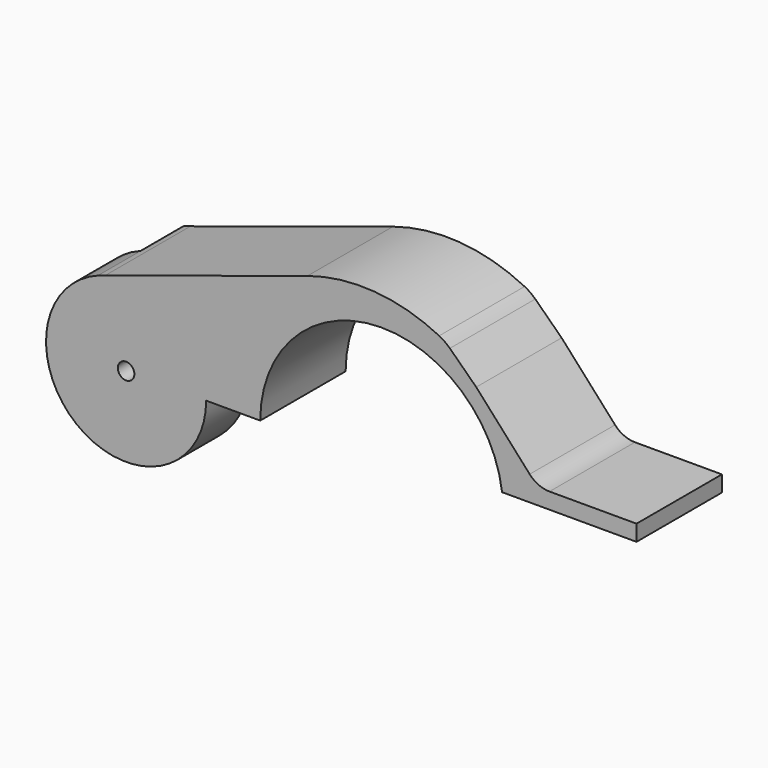
from build123d import *

# Parameters (mm, degrees)
F1_DEPTH = 20
F0_R     = 1.55
F2_DEPTH = 10


with BuildPart() as f1:
    # F0 (on Front) → F1 (new body)
    with BuildSketch(Plane.XZ):
        with BuildLine():
            ThreePointArc((-22.75, 0), (-1.4668388401, 22.702662483), (22.560846929, 2.9275733717))
            Line((22.560846929, 2.9275733717), (25.5830376256, 2.9275733717))
            Line((25.5830376256, 2.9275733717), (47.75, 2.9275733717))
            Line((47.75, 2.9275733717), (47.75, 5.9275733717))
            Line((47.75, 5.9275733717), (31.4456390027, 5.9275733717))
            ThreePointArc((31.4456390027, 5.9275733717), (29.4136159552, 6.3591072905), (27.7323476553, 7.5792204378))
            Line((27.7323476553, 7.5792204378), (17.7172674824, 18.6858484677))
            Line((17.7172674824, 18.6858484677), (12.7792477744, 23.4759662812))
            ThreePointArc((12.7792477744, 23.4759662812), (11.8349502961, 24.2607131327), (10.7816891456, 24.8917173301))
            ThreePointArc((10.7816891456, 24.8917173301), (-1.3748763237, 28.2426544781), (-13.8956863698, 26.7459315358))
            Line((-13.8956863698, 26.7459315358), (-51.8277890626, 14.4719109537))
            ThreePointArc((-51.8277890626, 14.4719109537), (-38.7771016598, 11.9200767766), (-32.8826916814, 0))
            Line((-32.8826916814, 0), (-25.75, 0))
            Line((-25.75, 0), (-22.75, 0))
        make_face()
    extrude(amount=-F1_DEPTH)

    # F0 (on Front) → F2 (join)
    with BuildSketch(Plane.XZ):
        with BuildLine():
            ThreePointArc((-53.1633601138, 14.0397486056), (-56.4205477798, -12.33308612), (-32.8826916814, 0))
            ThreePointArc((-32.8826916814, 0), (-38.7771016598, 11.9200767766), (-51.8277890626, 14.4719109537))
            Line((-51.8277890626, 14.4719109537), (-53.1633601138, 14.0397486056))
        make_face()
        with Locations((-47.8826916814, 0)):
            Circle(F0_R, mode=Mode.SUBTRACT)
    extrude(amount=-F2_DEPTH)


with BuildPart() as f1b:
    # F0 (on Front) → F1, piece 2 (new body)
    with BuildSketch(Plane.XZ):
        with BuildLine():
            ThreePointArc((-51.8277890626, 14.4719109537), (-52.5006327578, 14.2714617406), (-53.1633601138, 14.0397486056))
            Line((-53.1633601138, 14.0397486056), (-51.8277890626, 14.4719109537))
        make_face()
    extrude(amount=-F1_DEPTH)


solid = Compound([f1.part, f1b.part])
